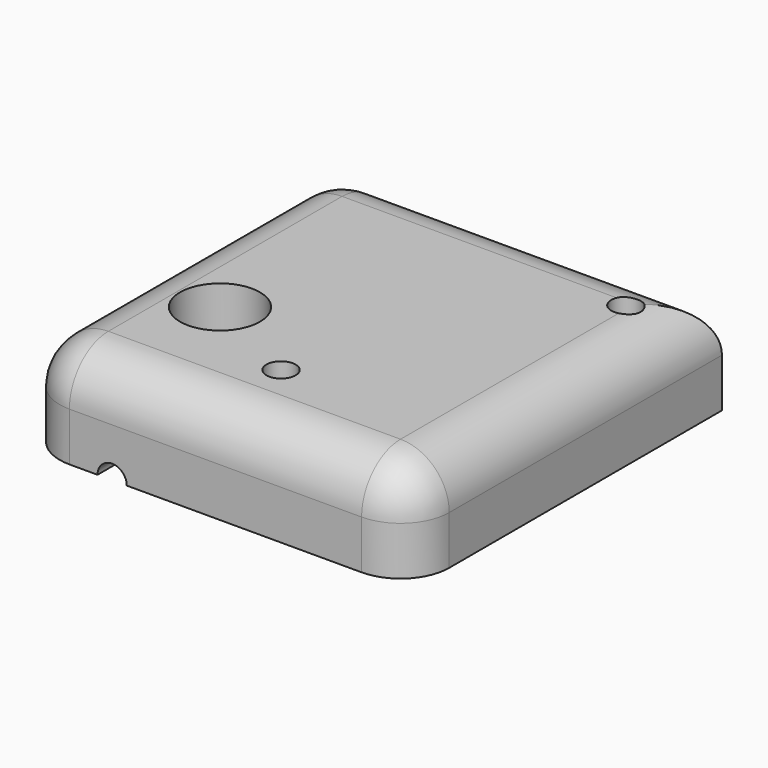
from build123d import *

# Parameters (mm, degrees)
F0_W          = 40
F0_H          = 40
F1_DEPTH      = 10
F3_DEPTH      = 0.5
F4_R          = 4.1
F5_DEPTH      = 10.001
F7_W          = 2.5
F7_H          = 2.75
F8_DEPTH      = 15
F11_REACH     = 43.3551019662
F12_R         = 1.5
F13_DEPTH     = 10.0010001
F14_T1_DEPTH  = 17.5
F14_T3_DEPTH  = 47.5
F14_T5_DEPTH  = 30
F14_T7_DEPTH  = 30
F14_T9_DEPTH  = 47.5
F14_S13_W     = 5
F14_S13_H     = 5
F14_T14_DEPTH = 5
F14_S19_W     = 5
F14_S19_H     = 5
F14_T20_DEPTH = 5
F14_S25_W     = 5
F14_S25_H     = 5
F14_T26_DEPTH = 5


# Not quite as in the source:
# - a fillet or chamfer that OpenCascade refuses, or shapes differently, is made with other operations: its cross-section is extruded or revolved along the edge and cut away or added


with BuildPart() as f1:
    # F0 (on Top) → F1 (new body)
    with BuildSketch(Plane.XY):
        Rectangle(F0_W, F0_H)
    extrude(amount=F1_DEPTH)

    # F2 (on face) → F3 (cut)
    with BuildSketch(Plane(origin=(0, 0, 0), x_dir=(1, 0, 0), z_dir=(0, 0, -1))):
        Polygon((11.3946354911, 9.8654455945), (-14.7593317032, -5.2345544055), (-14.7593317032, -20), (-5.3464073564, -20), (11.3946354911, -10.3345544055), align=None)
    extrude(amount=-F3_DEPTH, mode=Mode.SUBTRACT)

    # F4 (on face) → F5 (cut, through all)
    with BuildSketch(Plane(origin=(0, 0, 0), x_dir=(1, 0, 0), z_dir=(0, 0, -1))):
        with Locations((-10.6475949287, 6.1114258133)):
            Circle(F4_R)
    extrude(amount=-F5_DEPTH, mode=Mode.SUBTRACT)

    # F7 (on face) → F8 (cut)
    with BuildSketch(Plane(origin=(-20, 0, 0), x_dir=(0, -1, 0), z_dir=(-1, 0, 0))):
        with Locations((13.6307496577, 1.375)):
            Rectangle(F7_W, F7_H)
    extrude(amount=-F8_DEPTH, mode=Mode.SUBTRACT)

    f11_end = f1.faces().sort_by_distance((-14.7475949287, -6.1114258133, 5))[0]
    # F10 (on face) → F11 (cut, up to a face of the model that its end follows)
    with BuildSketch(Plane.XZ.offset(20)):
        with BuildLine():
            Line((-12.1130503118, 0), (-9.1130503118, 0))
            ThreePointArc((-9.1130503118, 0), (-10.6130503118, 1.5), (-12.1130503118, 0))
        make_face()
    f11_long = extrude(amount=-F11_REACH, mode=Mode.PRIVATE)
    add(split(f11_long, bisect_by=f11_end, keep=Keep.ALL, mode=Mode.PRIVATE).solids().sort_by_distance((-10.6130503118, -20, 0.6366197724))[0], mode=Mode.SUBTRACT)

    # F12 (on face) → F13 (cut, through all)
    with BuildSketch(Plane(origin=(0, 0, 0), x_dir=(1, 0, 0), z_dir=(0, 0, -1))):
        with Locations((0, 11.5903077688)):
            Circle(F12_R)
        with Locations((14.5839625479, -14.4456071497)):
            Circle(F12_R)
    extrude(amount=-F13_DEPTH, mode=Mode.SUBTRACT)

    # F14: fillet of radius 5 on 7 edges, made by hand

    # F14_s2 → F14_t1 (cut)
    with BuildSketch(Plane.XY.offset(-12.5)):
        with BuildLine():
            ThreePointArc((-15, -20), (-18.5355339059, -18.5355339059), (-20, -15))
            Line((-20, -15), (-20, -20))
            Line((-20, -20), (-15, -20))
        make_face()
        with BuildLine():
            ThreePointArc((-20, 15), (-18.5355339059, 18.5355339059), (-15, 20))
            Line((-15, 20), (-20, 20))
            Line((-20, 20), (-20, 15))
        make_face()
        with BuildLine():
            ThreePointArc((15, -20), (18.5355339059, -18.5355339059), (20, -15))
            Line((20, -15), (20, -20))
            Line((20, -20), (15, -20))
        make_face()
    extrude(amount=F14_T1_DEPTH, mode=Mode.SUBTRACT)

    # F14_s4 → F14_t3 (cut)
    with BuildSketch(Plane.XZ.offset(-32.5)):
        with BuildLine():
            ThreePointArc((20, 5), (18.5355339059, 8.5355339059), (15, 10))
            Line((15, 10), (20, 10))
            Line((20, 10), (20, 5))
        make_face()
    extrude(amount=F14_T3_DEPTH, mode=Mode.SUBTRACT)

    # F14_s6 → F14_t5 (cut)
    with BuildSketch(Plane.YZ.offset(-15)):
        with BuildLine():
            ThreePointArc((-20, 5), (-18.5355339059, 8.5355339059), (-15, 10))
            Line((-15, 10), (-20, 10))
            Line((-20, 10), (-20, 5))
        make_face()
    extrude(amount=F14_T5_DEPTH, mode=Mode.SUBTRACT)

    # F14_s8 → F14_t7 (cut)
    with BuildSketch(Plane.XZ.offset(-15)):
        with BuildLine():
            ThreePointArc((-15, 10), (-18.5355339059, 8.5355339059), (-20, 5))
            Line((-20, 5), (-20, 10))
            Line((-20, 10), (-15, 10))
        make_face()
    extrude(amount=F14_T7_DEPTH, mode=Mode.SUBTRACT)

    # F14_s10 → F14_t9 (cut)
    with BuildSketch(Plane.YZ.offset(-15)):
        with BuildLine():
            ThreePointArc((15, 10), (18.5355339059, 8.5355339059), (20, 5))
            Line((20, 5), (20, 10))
            Line((20, 10), (15, 10))
        make_face()
    extrude(amount=F14_T9_DEPTH, mode=Mode.SUBTRACT)


with BuildPart() as f14_tool12:
    # F14_s13 → F14_t14 (new body)
    with BuildSketch(Plane.XZ.offset(15)):
        with Locations((-17.5, 7.5)):
            Rectangle(F14_S13_W, F14_S13_H)
    extrude(amount=F14_T14_DEPTH)

    # F14_s15 → F14_t16 (revolve, cut)
    with BuildSketch(Plane(origin=(-15, -15, 5), x_dir=(0.7071067812, 0, -0.7071067812), z_dir=(-0.7071067812, 0, -0.7071067812))):
        with BuildLine():
            ThreePointArc((0, -5), (5, 0), (0, 5))
            Line((0, 5), (0, -5))
        make_face()
    revolve(axis=Axis((-15, -15, 5), (0, -1, 0)), mode=Mode.SUBTRACT)


with BuildPart() as f1_1:
    add(f1.part)

    # F14_t11: cut F14_tool12
    add(f14_tool12.part, mode=Mode.SUBTRACT)


with BuildPart() as f14_tool18:
    # F14_s19 → F14_t20 (new body)
    with BuildSketch(Plane.XZ.offset(-15)):
        with Locations((-17.5, 7.5)):
            Rectangle(F14_S19_W, F14_S19_H)
    extrude(amount=-F14_T20_DEPTH)

    # F14_s21 → F14_t22 (revolve, cut)
    with BuildSketch(Plane(origin=(-15, 15, 5), x_dir=(0.7071067812, 0, -0.7071067812), z_dir=(0.7071067812, 0, 0.7071067812))):
        with BuildLine():
            ThreePointArc((0, -5), (5, 0), (0, 5))
            Line((0, 5), (0, -5))
        make_face()
    revolve(axis=Axis((-15, 15, 5), (0, 1, 0)), mode=Mode.SUBTRACT)


with BuildPart() as f1_2:
    add(f1_1.part)

    # F14_t17: cut F14_tool18
    add(f14_tool18.part, mode=Mode.SUBTRACT)


with BuildPart() as f14_tool24:
    # F14_s25 → F14_t26 (new body)
    with BuildSketch(Plane.XZ.offset(15)):
        with Locations((17.5, 7.5)):
            Rectangle(F14_S25_W, F14_S25_H)
    extrude(amount=F14_T26_DEPTH)

    # F14_s27 → F14_t28 (revolve, cut)
    with BuildSketch(Plane(origin=(15, -15, 5), x_dir=(-0.7071067812, 0, -0.7071067812), z_dir=(-0.7071067812, 0, 0.7071067812))):
        with BuildLine():
            ThreePointArc((0, -5), (5, 0), (0, 5))
            Line((0, 5), (0, -5))
        make_face()
    revolve(axis=Axis((15, -15, 5), (0, -1, 0)), mode=Mode.SUBTRACT)


with BuildPart() as f1_3:
    add(f1_2.part)

    # F14_t23: cut F14_tool24
    add(f14_tool24.part, mode=Mode.SUBTRACT)


solid = f1_3.part
